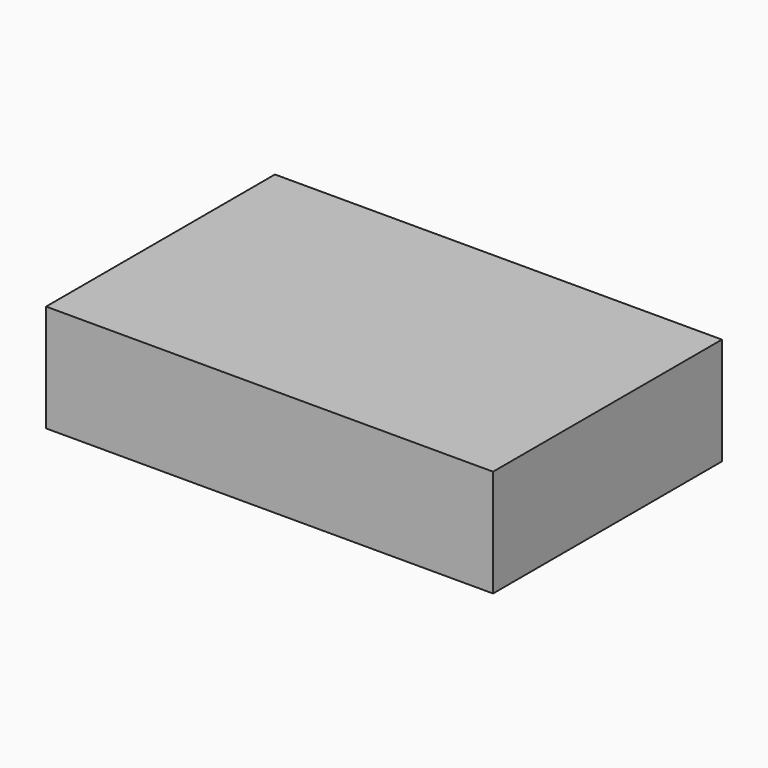
from build123d import *

# Parameters (mm, degrees)
F0_W     = 79.375
F0_H     = 50.8
F1_DEPTH = 19.05


# Not quite as in the source:
# - a length typed as a fraction of an inch, garbled in the dataset ("3 / 203.2 mm" for 3/8 in), is restored


with BuildPart() as f1:
    # F0 (on Top) → F1 (new body)
    with BuildSketch(Plane.XY):
        with Locations((39.6875, 25.4)):
            Rectangle(F0_W, F0_H)
    extrude(amount=F1_DEPTH)


solid = f1.part
